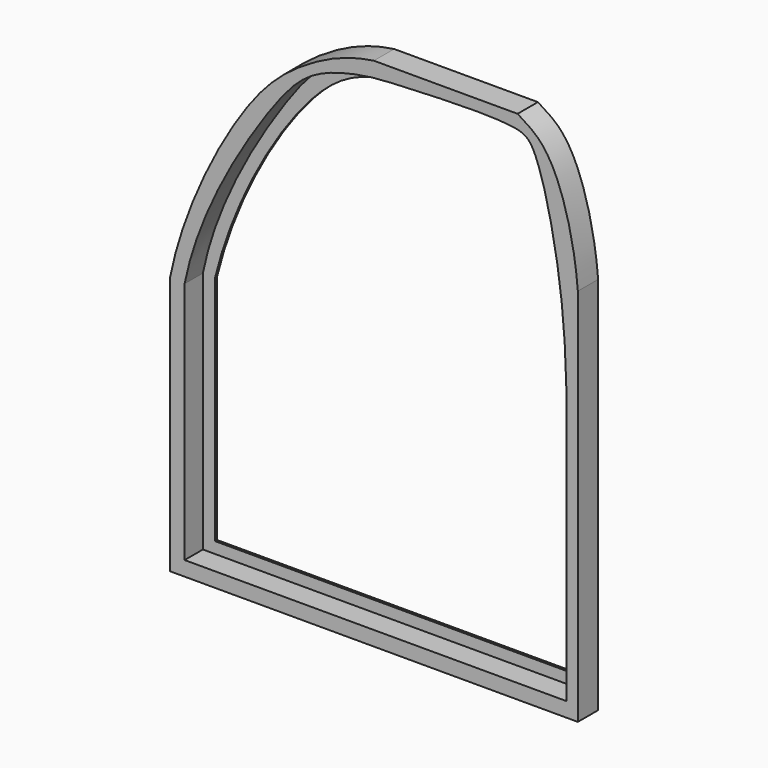
from build123d import *

# Parameters (mm, degrees)
F1_DEPTH = 5
F2_DEPTH = 0.5


with BuildPart() as f1:
    # F0 (on Front) → F1 (new body)
    with BuildSketch(Plane.XZ):
        with BuildLine():
            Line((21.9498877709, 46.5069999899), (-6.3801594079, 46.5069999899))
            add(Edge.make_bspline(
                [(-46.5855710208, -4.3176412582), (-44.0025745855, 8.8650835819), (-32.3669471438, 31.5826223404), (-20.8450996019, 41.430559805), (-11.9788710798, 45.7277535437), (-6.3801594079, 46.5069999899)],
                knots=[0, 0, 0, 0, 0.4471722481, 0.7226417186, 1, 1, 1, 1], degree=3))
            Line((-46.5855710208, -4.3176412582), (-46.5855710208, -55.1422825063))
            Line((-46.5855710208, -55.1422825063), (33.8252522051, -55.1422825063))
            Line((33.8252522051, -55.1422825063), (33.8252522051, 3.3716567512))
            add(Edge.make_bspline(
                [(33.8252522051, 3.4864664458), (33.8224510146, 3.4189701607), (33.823496077, 3.4012213221), (33.8252522051, 3.3716567512)],
                knots=[0.9714616128, 0.9714616128, 0.9714616128, 0.9714616128, 1, 1, 1, 1], degree=3))
            Line((33.8252522051, 3.4864664458), (33.8252522051, 19.6025110781))
            add(Edge.make_bspline(
                [(21.9498877709, 46.5069999899), (23.8964492564, 45.3404017708), (29.3341911452, 42.1357952335), (33.1026848595, 28.5809846581), (33.8252522051, 19.6025110781)],
                knots=[0, 0, 0, 0, 0.2303722913, 0.6333427683, 0.6333427683, 0.6333427683, 0.6333427683], degree=3))
        make_face()
        with BuildLine():
            Line((31.6210500896, -52.260261029), (-43.6766035855, -52.260261029))
            Line((-43.6766035855, -52.260261029), (-43.6766035855, -4.3176412582))
            add(Edge.make_bspline(
                [(-43.6766035855, -4.3176412582), (-41.0383021138, 9.0666906176), (-27.9398807539, 30.9156219348), (-18.7479844266, 41.3390835094), (-7.0085331076, 43.5985571671), (-2.215007715, 43.8020735184), (21.2993443911, 44.9657713637), (26.0800513958, 41.7197839808), (31.3102526714, 18.3624746495), (31.5930695379, 3.1075431018), (31.6210500896, -4.3176412582)],
                knots=[0, 0, 0, 0, 0.1942047864, 0.3092342936, 0.40822929, 0.4837495286, 0.6306580628, 0.7017097882, 0.8479049191, 1, 1, 1, 1], degree=3))
            Line((31.6210500896, -4.3176412582), (31.6210500896, -52.260261029))
        make_face(mode=Mode.SUBTRACT)
        with BuildLine():
            Line((33.8252522051, 3.3716567512), (33.8252522051, 3.4864664458))
            add(Edge.make_bspline(
                [(33.8252522051, 3.4864664458), (33.8224510146, 3.4189701607), (33.823496077, 3.4012213221), (33.8252522051, 3.3716567512)],
                knots=[0.9714616128, 0.9714616128, 0.9714616128, 0.9714616128, 1, 1, 1, 1], degree=3))
        make_face()
    extrude(amount=F1_DEPTH)

    # F0 (on Front) → F2 (join)
    with BuildSketch(Plane.XZ):
        with BuildLine():
            Line((-43.6766035855, -4.3176412582), (-43.6766035855, -52.260261029))
            Line((-43.6766035855, -52.260261029), (31.6210500896, -52.260261029))
            Line((31.6210500896, -52.260261029), (31.6210500896, -4.3176412582))
            add(Edge.make_bspline(
                [(-43.6766035855, -4.3176412582), (-41.0383021138, 9.0666906176), (-27.9398807539, 30.9156219348), (-18.7479844266, 41.3390835094), (-7.0085331076, 43.5985571671), (-2.215007715, 43.8020735184), (21.2993443911, 44.9657713637), (26.0800513958, 41.7197839808), (31.3102526714, 18.3624746495), (31.5930695379, 3.1075431018), (31.6210500896, -4.3176412582)],
                knots=[0, 0, 0, 0, 0.1942047864, 0.3092342936, 0.40822929, 0.4837495286, 0.6306580628, 0.7017097882, 0.8479049191, 1, 1, 1, 1], degree=3))
        make_face()
        with BuildLine():
            Line((29.4725894928, -50.028309226), (-41.2763357162, -50.028309226))
            Line((-41.2763357162, -50.028309226), (-41.2763357162, -4.3176412582))
            add(Edge.make_bspline(
                [(29.4725894928, -4.3176412582), (29.1241496967, 2.9787885737), (28.5454511929, 18.1687452905), (23.4164160844, 41.9172876242), (16.665337298, 42.2003372333), (-7.4096989865, 42.5160002908), (-22.9090094529, 36.1722681351), (-37.4855825891, 11.2133633357), (-41.2763357162, -4.3176412582)],
                knots=[0, 0, 0, 0, 0.1793175303, 0.3494515687, 0.4340680096, 0.6090858367, 0.7583926872, 1, 1, 1, 1], degree=3))
            Line((29.4725894928, -4.3176412582), (29.4725894928, -50.028309226))
        make_face(mode=Mode.SUBTRACT)
    extrude(amount=F2_DEPTH)


solid = f1.part
